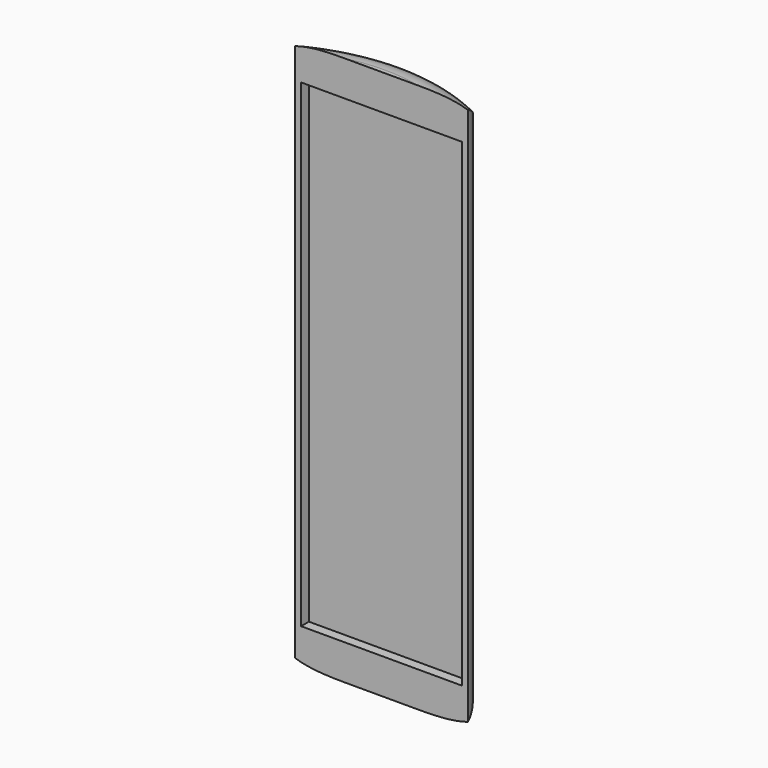
from build123d import *

# Parameters (mm, degrees)
F0_W        = 440
F0_H        = 40
F1_DEPTH    = 700
F2_W        = 410
F2_H        = 1220
F3_DEPTH    = 25
F4_T1_DEPTH = 1682.091793836
F4_T4_ANGLE = 98.0505806866
F4_T6_ANGLE = 98.0505806866


# Not quite as in the source:
# - a fillet or chamfer that OpenCascade refuses, or shapes differently, is made with other operations: its cross-section is extruded or revolved along the edge and cut away or added


with BuildPart() as f1:
    # F0 (on Top) → F1 (new body, symmetric)
    with BuildSketch(Plane.XY):
        Rectangle(F0_W, F0_H)
        with BuildLine():
            Line((-220, 20), (220, 20))
            ThreePointArc((220, 20), (0, 71.0011135871), (-220, 20))
        make_face()
    extrude(amount=F1_DEPTH, both=True)

    # F2 (on face) → F3 (cut)
    with BuildSketch(Plane.XZ.offset(20)):
        Rectangle(F2_W, F2_H)
    extrude(amount=-F3_DEPTH, mode=Mode.SUBTRACT)

    # F4: fillet of radius 80 on 4 edges, made by hand

    # F4_s2 → F4_t1 (cut)
    with BuildSketch(Plane.XY.offset(-841.045896918)):
        with BuildLine():
            ThreePointArc((220, -20), (202.4071901909, 18.0134665716), (168.0166018628, 41.9261835277))
            ThreePointArc((168.0166018628, 41.9261835277), (194.3178072419, 31.696880649), (220, 20))
            Line((220, 20), (220, -20))
        make_face()
        with BuildLine():
            ThreePointArc((-220, -20), (-202.4071901909, 18.0134665716), (-168.0166018628, 41.9261835277))
            ThreePointArc((-168.0166018628, 41.9261835277), (-194.3178072419, 31.696880649), (-220, 20))
            Line((-220, 20), (-220, -20))
        make_face()
    extrude(amount=F4_T1_DEPTH, mode=Mode.SUBTRACT)

    # F4_s3 → F4_t4 (revolve, cut)
    with BuildSketch(Plane(origin=(212.3855127845, -244.5395013814, 0), x_dir=(0, 0, 1), z_dir=(0.6557258365, -0.754999091, 0))):
        with BuildLine():
            ThreePointArc((700, -138.6943463652), (676.5685424949, -195.2628888601), (620, -218.6943463652))
            Line((620, -218.6943463652), (700, -218.6943463652))
            Line((700, -218.6943463652), (700, -138.6943463652))
        make_face()
    revolve(axis=Axis((0, -428.9988864129, 700), (0, 0, 1)), revolution_arc=F4_T4_ANGLE, mode=Mode.SUBTRACT)

    # F4_s5 → F4_t6 (revolve, cut)
    with BuildSketch(Plane(origin=(212.3855127845, -244.5395013814, 0), x_dir=(0, 0, 1), z_dir=(0.6557258365, -0.754999091, 0))):
        with BuildLine():
            ThreePointArc((-700, -138.6943463652), (-676.5685424949, -195.2628888601), (-620, -218.6943463652))
            Line((-620, -218.6943463652), (-700, -218.6943463652))
            Line((-700, -218.6943463652), (-700, -138.6943463652))
        make_face()
    revolve(axis=Axis((0, -428.9988864129, -700), (0, 0, 1)), revolution_arc=F4_T6_ANGLE, mode=Mode.SUBTRACT)


solid = f1.part
